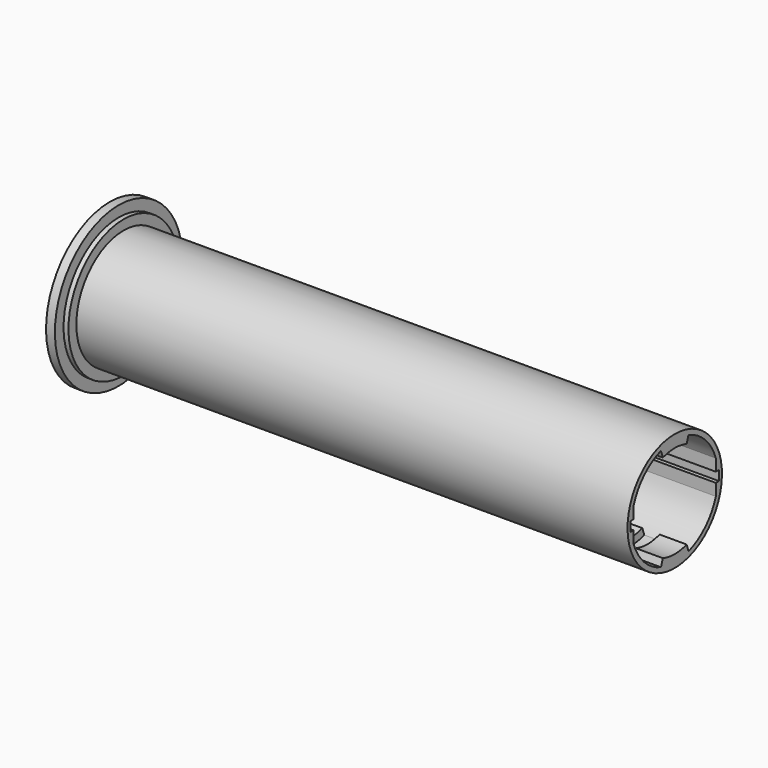
from build123d import *

# Parameters (mm, degrees)
F3_DEPTH        = 112
F4_R            = 12
F5_DEPTH        = 112.5
F7_DEPTH        = 3
F9_DEPTH        = 2
F9_COPIES_COUNT = 6
F11_START       = 57.5
F10_R           = 11
F11_DEPTH       = 3.5
F12_DEPTH       = 100


# Not quite as in the source:
# - a pattern or mirror of a feature is missing from the dataset's text; its kind, count and spacing are read off the source's solid


with BuildPart() as f1:
    # F0 (on Front) → F1 (revolve)
    with BuildSketch(Plane.XZ):
        Polygon((-50, 13.2), (-50, 0), (-46, 0), (-46, 11), (66.5, 11), (66.5, 12), (-45.6, 12), (-45.6, 14), (-46.6, 14), (-46.6, 16.2), (-48.4, 16.2), align=None)
    revolve(axis=Axis((3.169978948, 0, 0), (1, 0, 0)))

    # F2 (on face) → F3 (cut)
    with BuildSketch(Plane.YZ.offset(66.5)):
        with BuildLine():
            ThreePointArc((-10.9544511501, -1), (-11, 0), (-10.9544511501, 1))
            Line((-10.9544511501, 1), (-11.25, 1))
            Line((-11.25, 1), (-11.25, -1))
            Line((-11.25, -1), (-10.9544511501, -1))
        make_face()
        with BuildLine():
            Line((11.25, 1), (10.9544511501, 1))
            ThreePointArc((10.9544511501, 1), (10.9886068874, 0.5005184057), (11, 0))
            ThreePointArc((11, 0), (10.9886068874, -0.5005184057), (10.9544511501, -1))
            Line((10.9544511501, -1), (11.25, -1))
            Line((11.25, -1), (11.25, 1))
        make_face()
    extrude(amount=-F3_DEPTH, mode=Mode.SUBTRACT)

    # F4 (on face) → F5 (join, through all)
    with BuildSketch(Plane.YZ.offset(66.5)):
        Circle(F4_R)
        with BuildLine():
            ThreePointArc((-10.4544511501, 3.4211768662), (-7.8074781011, 7.7487602686), (-3.5, 10.4283268073))
            ThreePointArc((-3.5, 10.4283268073), (0, 11), (3.5, 10.4283268073))
            ThreePointArc((3.5, 10.4283268073), (7.8074781011, 7.7487602686), (10.4544511501, 3.4211768662))
            ThreePointArc((10.4544511501, 3.4211768662), (10.7726876303, 2.2246800266), (10.9544511501, 1))
            Line((10.9544511501, 1), (11.25, 1))
            Line((11.25, 1), (11.25, -1))
            Line((11.25, -1), (10.9544511501, -1))
            ThreePointArc((10.9544511501, -1), (10.7726876303, -2.2246800266), (10.4544511501, -3.4211768662))
            ThreePointArc((10.4544511501, -3.4211768662), (7.8074781011, -7.7487602686), (3.5, -10.4283268073))
            ThreePointArc((3.5, -10.4283268073), (0, -11), (-3.5, -10.4283268073))
            ThreePointArc((-3.5, -10.4283268073), (-7.8074781011, -7.7487602686), (-10.4544511501, -3.4211768662))
            ThreePointArc((-10.4544511501, -3.4211768662), (-10.7726876303, -2.2246800266), (-10.9544511501, -1))
            Line((-10.9544511501, -1), (-11.25, -1))
            Line((-11.25, -1), (-11.25, 1))
            Line((-11.25, 1), (-10.9544511501, 1))
            ThreePointArc((-10.9544511501, 1), (-10.7726876303, 2.2246800266), (-10.4544511501, 3.4211768662))
        make_face(mode=Mode.SUBTRACT)
        with BuildLine():
            ThreePointArc((3.5, 10.4283268073), (0, 11), (-3.5, 10.4283268073))
            Line((-3.5, 10.4283268073), (-3.0227272727, 9.0062822427))
            ThreePointArc((-3.0227272727, 9.0062822427), (0, 9.5), (3.0227272727, 9.0062822427))
            Line((3.0227272727, 9.0062822427), (3.5, 10.4283268073))
        make_face()
        with BuildLine():
            Line((-3.0227272727, -9.0062822427), (-3.5, -10.4283268073))
            ThreePointArc((-3.5, -10.4283268073), (0, -11), (3.5, -10.4283268073))
            Line((3.5, -10.4283268073), (3.0227272727, -9.0062822427))
            ThreePointArc((3.0227272727, -9.0062822427), (0, -9.5), (-3.0227272727, -9.0062822427))
        make_face()
    extrude(amount=-F5_DEPTH)

    # F6 (on face) → F7 (cut)
    with BuildSketch(Plane(origin=(-50, 0, 0), x_dir=(0, -1, 0), z_dir=(-1, 0, 0))):
        Polygon((-4.3301270189, 0), (-2.1650635095, -3.75), (2.1650635095, -3.75), (4.3301270189, 0), (2.1650635095, 3.75), (-2.1650635095, 3.75), align=None)
    extrude(amount=-F7_DEPTH, mode=Mode.SUBTRACT)

    # F8 (on face) → F9 (cut)
    with BuildSketch(Plane(origin=(-50, 0, 0), x_dir=(0, -1, 0), z_dir=(-1, 0, 0))):
        with BuildLine():
            Line((1.5, 15), (-1.5, 15))
            Line((-1.5, 15), (-1.5, 12.5))
            ThreePointArc((-1.5, 12.5), (0, 11), (1.5, 12.5))
            Line((1.5, 12.5), (1.5, 15))
        make_face()
    f9 = extrude(amount=-F9_DEPTH, mode=Mode.SUBTRACT)

    # F9_copies: F9 ×6 about axis
    f9_copies_axis = Axis((0, 0, 0), (1, 0, 0))
    for i in range(1, F9_COPIES_COUNT):
        add(f9.rotate(f9_copies_axis, i * 360 / F9_COPIES_COUNT), mode=Mode.SUBTRACT)

    # F10 (on Right) → F11 (cut)
    with BuildSketch(Plane.YZ.offset(F11_START)):
        Circle(F10_R)
    extrude(amount=F11_DEPTH, mode=Mode.SUBTRACT)

    # F2 (on face) → F12 (join)
    with BuildSketch(Plane.YZ.offset(66.5)):
        with BuildLine():
            Line((10.4544511501, 1), (10.9544511501, 1))
            ThreePointArc((10.9544511501, 1), (10.7726876303, 2.2246800266), (10.4544511501, 3.4211768662))
            Line((10.4544511501, 3.4211768662), (10.4544511501, 1))
        make_face()
        with BuildLine():
            ThreePointArc((10.4544511501, -3.4211768662), (10.7726876303, -2.2246800266), (10.9544511501, -1))
            Line((10.9544511501, -1), (10.4544511501, -1))
            Line((10.4544511501, -1), (10.4544511501, -3.4211768662))
        make_face()
        with BuildLine():
            ThreePointArc((-10.9544511501, -1), (-10.7726876303, -2.2246800266), (-10.4544511501, -3.4211768662))
            Line((-10.4544511501, -3.4211768662), (-10.4544511501, -1))
            Line((-10.4544511501, -1), (-10.9544511501, -1))
        make_face()
        with BuildLine():
            Line((-10.4544511501, 1), (-10.4544511501, 3.4211768662))
            ThreePointArc((-10.4544511501, 3.4211768662), (-10.7726876303, 2.2246800266), (-10.9544511501, 1))
            Line((-10.9544511501, 1), (-10.4544511501, 1))
        make_face()
    extrude(amount=-F12_DEPTH)


solid = f1.part
